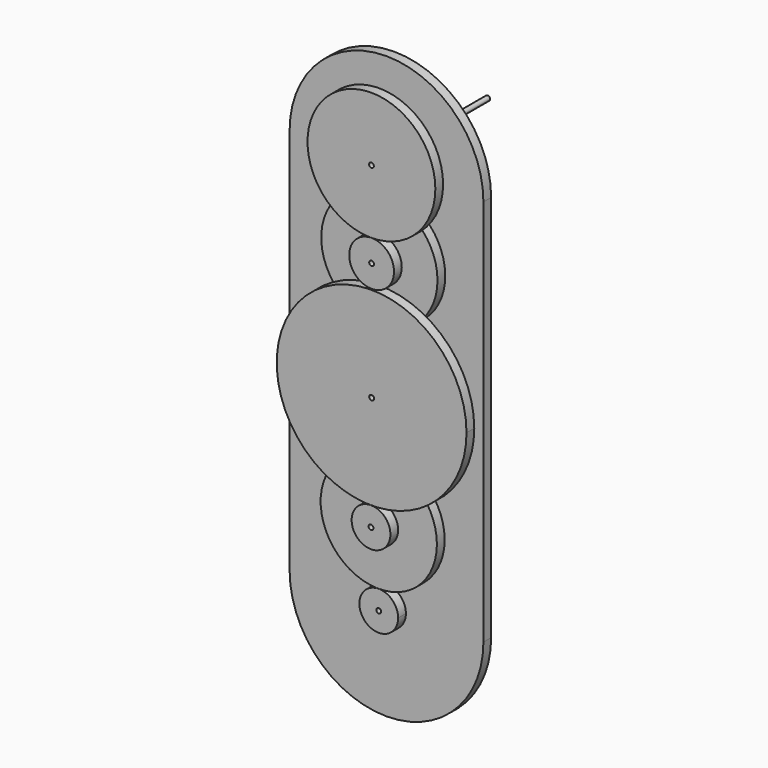
from build123d import *

# Parameters (mm, degrees)
F0_W      = 127
F0_H      = 254
F1_DEPTH  = 6.35
F4_DEPTH  = 6.35
F5_R      = 12.7
F6_DEPTH  = 6.35
F8_DEPTH  = 6.35
F10_DEPTH = 6.35
F11_R     = 14.6844956333
F12_DEPTH = 6.35
F14_DEPTH = 6.35
F15_R     = 41.8862190393
F16_DEPTH = 6.35
F17_R     = 1.5875
F18_DEPTH = 19.051
F19_DEPTH = 76.2


# Not quite as in the source:
# - the program builds the solid bodies; features that only make, move or delete a surface that nothing else refers to are left out


with BuildPart() as f1:
    # F0 (on Front) → F1 (new body)
    with BuildSketch(Plane.XZ):
        with Locations((63.5, 127)):
            Rectangle(F0_W, F0_H)
        with BuildLine():
            ThreePointArc((127, 254), (63.5, 317.5), (0, 254))
            Line((0, 254), (127, 254))
        make_face()
        with BuildLine():
            Line((127, 0), (0, 0))
            ThreePointArc((0, 0), (63.5, -63.5), (127, 0))
        make_face()
    extrude(amount=F1_DEPTH)


with BuildPart() as f4:
    # F2 (on face) → F4 (new body)
    with BuildSketch(Plane.XZ.offset(6.35)):
        with BuildLine():
            ThreePointArc((63.5, 88.9), (25.4, 50.7999999784), (63.5000000432, 12.7))
            ThreePointArc((63.5000000432, 12.7), (90.4407683785, 23.8592316521), (101.6, 50.8))
            ThreePointArc((101.6, 50.8), (90.4407683632, 77.7407683632), (63.5, 88.9))
        make_face()
    extrude(amount=F4_DEPTH)


with BuildPart() as f4b:
    # F2 (on face) → F4, piece 2 (new body)
    with BuildSketch(Plane.XZ.offset(6.35)):
        with BuildLine():
            ThreePointArc((63.5000000432, 12.7), (54.5197438636, -8.9802561058), (76.2, 0))
            ThreePointArc((76.2, 0), (72.4802561364, 8.9802561058), (63.5000000432, 12.7))
        make_face()
    extrude(amount=F4_DEPTH)


with BuildPart() as f6:
    # F5 (on face) → F6 (new body)
    with BuildSketch(Plane.XZ.offset(12.7)):
        with Locations((63.5, 50.8)):
            Circle(F5_R)
    extrude(amount=F6_DEPTH)


with BuildPart() as f8:
    # F7 (on face) → F8 (new body)
    with BuildSketch(Plane.XZ.offset(12.7)):
        with BuildLine():
            ThreePointArc((95.1926497876, 71.946771608), (63.7019956295, 88.8994645338), (32.0333573438, 72.2816293597))
            ThreePointArc((32.0333573438, 72.2816293597), (63.5673318765, 63.4998215113), (95.1926497876, 71.946771608))
        make_face()
        with BuildLine():
            ThreePointArc((95.1926497876, 71.946771608), (117.8147364594, 94.69498662), (126.0893906907, 125.6912797689))
            ThreePointArc((126.0893906907, 125.6912797689), (33.1870574181, 179.7725338358), (32.0333573438, 72.2816293597))
            ThreePointArc((32.0333573438, 72.2816293597), (63.7019956295, 88.8994645338), (95.1926497876, 71.946771608))
        make_face()
    extrude(amount=F8_DEPTH)


with BuildPart() as f10:
    # F3 (on face) → F10 (new body)
    with BuildSketch(Plane.XZ.offset(6.35)):
        with BuildLine():
            ThreePointArc((63.6960125926, 165.0994957849), (90.7634033509, 176.1890111487), (101.9920253124, 203.1989915691))
            ThreePointArc((101.9920253124, 203.1989915691), (37.020647274, 230.2089719896), (63.6960125926, 165.0994957849))
        make_face()
    extrude(amount=F10_DEPTH)

    # F11 (on face) → F12 (join)
    with BuildSketch(Plane.XZ.offset(12.7)):
        with Locations((63.8920253124, 203.1989915691)):
            Circle(F11_R)
    extrude(amount=F12_DEPTH)


with BuildPart() as f14:
    # F13 (on face) → F14 (new body)
    with BuildSketch(Plane.XZ.offset(6.35)):
        with BuildLine():
            ThreePointArc((76.4929108533, 259.7695887089), (63.7767091393, 272.4857904229), (51.0605074254, 259.7695887089))
            Line((51.0605074254, 259.7695887089), (76.4929108533, 259.7695887089))
        make_face()
        with BuildLine():
            Line((76.4929108533, 259.7695887089), (51.0605074254, 259.7695887089))
            ThreePointArc((51.0605074254, 259.7695887089), (63.7767091393, 247.0533869949), (76.4929108533, 259.7695887089))
        make_face()
    extrude(amount=F14_DEPTH)


with BuildPart() as f16:
    # F15 (on face) → F16 (new body)
    with BuildSketch(Plane.XZ.offset(12.7)):
        with Locations((63.7767091393, 259.7695887089)):
            Circle(F15_R)
    extrude(amount=F16_DEPTH)


with BuildPart() as f18_tool:
    # F17 (on face) → F18 (new body, through all)
    with BuildSketch(Plane(origin=(0, 0, 0), x_dir=(-1, 0, 0), z_dir=(0, 1, 0))):
        with Locations((-63.7767091393, 259.7695887089)):
            Circle(F17_R)
        with Locations((-63.8920253124, 203.1989915691)):
            Circle(F17_R)
        with Locations((-63.8970583677, 125.6912797689)):
            Circle(F17_R)
        with Locations((-63.5, 50.8)):
            Circle(F17_R)
        with Locations((-63.5, 0)):
            Circle(F17_R)
    extrude(amount=-F18_DEPTH)


with BuildPart() as f1_1:
    add(f1.part)

    # F18: cut by f18_tool
    add(f18_tool.part, mode=Mode.SUBTRACT)


with BuildPart() as f4_1:
    add(f4.part)

    # F18: cut by f18_tool
    add(f18_tool.part, mode=Mode.SUBTRACT)


with BuildPart() as f4b_1:
    add(f4b.part)

    # F18: cut by f18_tool
    add(f18_tool.part, mode=Mode.SUBTRACT)


with BuildPart() as f6_1:
    add(f6.part)

    # F18: cut by f18_tool
    add(f18_tool.part, mode=Mode.SUBTRACT)


with BuildPart() as f8_1:
    add(f8.part)

    # F18: cut by f18_tool
    add(f18_tool.part, mode=Mode.SUBTRACT)


with BuildPart() as f10_1:
    add(f10.part)

    # F18: cut by f18_tool
    add(f18_tool.part, mode=Mode.SUBTRACT)


with BuildPart() as f14_1:
    add(f14.part)

    # F18: cut by f18_tool
    add(f18_tool.part, mode=Mode.SUBTRACT)


with BuildPart() as f16_1:
    add(f16.part)

    # F18: cut by f18_tool
    add(f18_tool.part, mode=Mode.SUBTRACT)


with BuildPart() as f19:
    # F17 (on face) → F19 (new body)
    with BuildSketch(Plane(origin=(0, 0, 0), x_dir=(-1, 0, 0), z_dir=(0, 1, 0))):
        with Locations((-63.7767091393, 259.7695887089)):
            Circle(F17_R)
    extrude(amount=F19_DEPTH)


solid = Compound([f1_1.part, f4_1.part, f4b_1.part, f6_1.part, f8_1.part, f10_1.part, f14_1.part, f16_1.part, f19.part])
